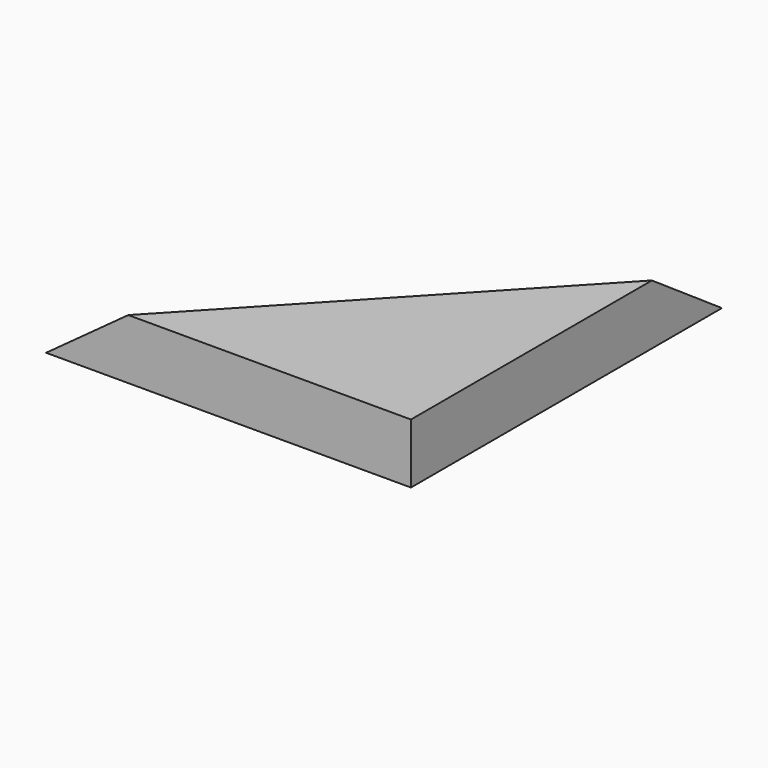
from build123d import *

# Parameters (mm, degrees)
F2_DEPTH = 12.446
F3_SIZE  = 12.44599


# Not quite as in the source:
# - a fillet or chamfer is up to 0.001 mm smaller than in the source, because OpenCascade refuses the exact size


with BuildPart() as f2:
    # F1 (on face) → F2 (new body)
    with BuildSketch(Plane.XY):
        Polygon((-75.7983550429, 29.4131990522), (0, 29.4131990522), (0, 110.1594716311), align=None)
    extrude(amount=F2_DEPTH)

    # F3 (size 12.446 in the source; OpenCascade refuses exactly that, so slightly less here)
    f3_edges = [f2.edges().sort_by_distance(p)[0] for p in [
        (-37.899178, 69.786335, 12.446),
    ]]
    chamfer(f3_edges, length=F3_SIZE)


solid = f2.part
